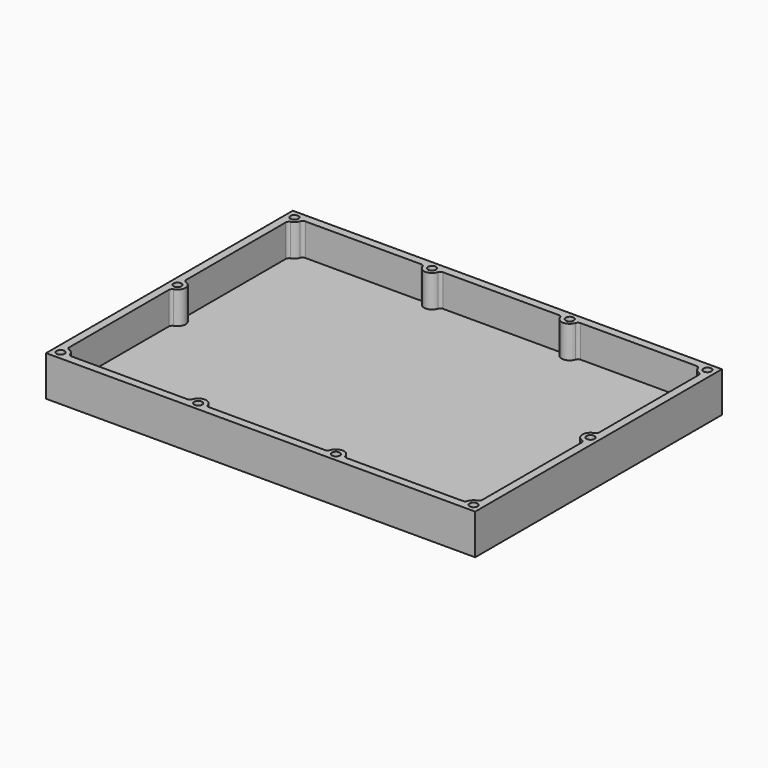
from build123d import *

# Parameters (mm, degrees)
F0_W             = 81.28
F0_H             = 58.42
F1_DEPTH         = 3.81
F2_T             = -1.524
F4_DEPTH         = 6.096
F4_COPIES2_COUNT = 2
F6_D             = 1.5113
F6_DEPTH         = 4.826
F6_TIP           = 0.4540403268
F7_R             = 0.635


# Not quite as in the source:
# - a pattern or mirror of a feature is missing from the dataset's text; its kind, count and spacing are read off the source's solid


with BuildPart() as f1:
    # F0 (on Top) → F1 (new body, symmetric)
    with BuildSketch(Plane.XY):
        Rectangle(F0_W, F0_H)
    extrude(amount=F1_DEPTH, both=True)

    # F2
    f2_openings = [f1.faces().sort_by_distance(p)[0] for p in [
        (0, 0, 3.81),
    ]]
    offset(amount=F2_T, openings=f2_openings)

    # F3 (on face) → F4 (join, through all)
    with BuildSketch(Plane.XY.offset(3.81)):
        with BuildLine():
            ThreePointArc((-39.116, 26.162), (-38.0383692655, 26.6083692655), (-37.592, 27.686))
            Line((-37.592, 27.686), (-39.116, 27.686))
            Line((-39.116, 27.686), (-39.116, 26.162))
        make_face()
        with BuildLine():
            ThreePointArc((-13.0386666835, 29.21), (-14.1162974072, 28.7636307286), (-14.5626666667, 27.686))
            Line((-14.5626666667, 27.686), (-11.5146666667, 27.686))
            ThreePointArc((-11.5146666667, 27.686), (-11.9610359381, 28.7636307405), (-13.0386666835, 29.21))
        make_face()
        with BuildLine():
            Line((-39.116, -1.524), (-39.116, 1.524))
            ThreePointArc((-39.116, 1.524), (-40.1936307323, 1.0776307368), (-40.64, 6.4e-09))
            ThreePointArc((-40.64, 6.4e-09), (-40.1936307368, -1.0776307323), (-39.116, -1.524))
        make_face()
        with BuildLine():
            ThreePointArc((14.5626666667, 27.686), (14.1162974012, 28.7636307345), (13.0386666667, 29.21))
            ThreePointArc((13.0386666667, 29.21), (11.9610359321, 28.7636307345), (11.5146666667, 27.686))
            Line((11.5146666667, 27.686), (14.5626666667, 27.686))
        make_face()
        with BuildLine():
            Line((14.5626666667, 27.686), (11.5146666667, 27.686))
            ThreePointArc((11.5146666667, 27.686), (13.0386666667, 26.162), (14.5626666667, 27.686))
        make_face()
        with BuildLine():
            ThreePointArc((-37.592, -27.686), (-38.0383692655, -26.6083692655), (-39.116, -26.162))
            Line((-39.116, -26.162), (-39.116, -27.686))
            Line((-39.116, -27.686), (-37.592, -27.686))
        make_face()
        with BuildLine():
            Line((39.116, 27.686), (37.592, 27.686))
            ThreePointArc((37.592, 27.686), (38.0383692655, 26.6083692655), (39.116, 26.162))
            Line((39.116, 26.162), (39.116, 27.686))
        make_face()
        with BuildLine():
            ThreePointArc((-14.5626666667, -27.686), (-14.1162973989, -28.7636307368), (-13.0386666602, -29.21))
            ThreePointArc((-13.0386666602, -29.21), (-11.9610359299, -28.7636307323), (-11.5146666667, -27.686))
            Line((-11.5146666667, -27.686), (-14.5626666667, -27.686))
        make_face()
        with BuildLine():
            ThreePointArc((11.5146666667, -27.686), (11.9610359295, -28.7636307319), (13.0386666593, -29.21))
            ThreePointArc((13.0386666593, -29.21), (14.1162973986, -28.7636307371), (14.5626666667, -27.686))
            Line((14.5626666667, -27.686), (11.5146666667, -27.686))
        make_face()
        with BuildLine():
            Line((39.116, -1.524), (39.116, 1.524))
            ThreePointArc((39.116, 1.524), (37.592, 0), (39.116, -1.524))
        make_face()
        with BuildLine():
            Line((39.116, -27.686), (39.116, -26.162))
            ThreePointArc((39.116, -26.162), (38.0383692655, -26.6083692655), (37.592, -27.686))
            Line((37.592, -27.686), (39.116, -27.686))
        make_face()
    f4 = extrude(amount=-F4_DEPTH)

    # F4_copies: F4 across plane
    add(f4.mirror(Plane(origin=(0, 0, 0), x_dir=(0, 0, -1), z_dir=(-1, 0, 0))))

    # F4_copies1: F4 across plane
    add(f4.mirror(Plane(origin=(0, 0, 0), x_dir=(0, 0, -1), z_dir=(0, -1, 0))))

    # F4_copies2: F4 ×2 about axis
    f4_copies2_axis = Axis((0, 0, 0), (0, 0, 1))
    for i in range(1, F4_COPIES2_COUNT):
        add(f4.rotate(f4_copies2_axis, i * 360 / F4_COPIES2_COUNT))

    # F6
    with Locations(Plane.XY.offset(3.81)):
        with Locations((-39.116, 27.686), (-13.0386666667, 27.686), (13.0386666667, 27.686), (39.116, 27.686), (39.116, 0), (39.116, -27.686), (13.0386666667, -27.686), (-13.0386666667, -27.686), (-39.116, -27.686), (-39.116, 0)):
            Hole(F6_D / 2, depth=F6_DEPTH)
            with Locations((0, 0, -(F6_DEPTH + F6_TIP / 2))):  # 118° drill point
                Cone(0, F6_D / 2, F6_TIP, mode=Mode.SUBTRACT)

    # F7
    f7_edges = [f1.edges().sort_by_distance(p)[0] for p in [
        (-37.592, 27.686, 0.762),
        (-11.514667, 27.686, 0.762),
        (14.562667, 27.686, 0.762),
        (37.592, 27.686, 0.762),
        (40.64, 0, 0.762),
        (39.116, -26.162, 0.762),
        (37.592, -27.686, 0.762),
        (14.562667, -27.686, 0.762),
        (-11.514667, -27.686, 0.762),
        (-37.592, -27.686, 0.762),
        (39.116, 26.162, 0.762),
        (39.116, 1.524, 0.762),
        (39.116, -1.524, 0.762),
        (11.514667, 27.686, 0.762),
        (11.514667, -27.686, 0.762),
        (-14.562667, 27.686, 0.762),
        (-14.562667, -27.686, 0.762),
        (-39.116, 26.162, 0.762),
        (-39.116, 1.524, 0.762),
        (-39.116, -26.162, 0.762),
        (-39.116, -1.524, 0.762),
    ]]
    fillet(f7_edges, radius=F7_R)


solid = f1.part
